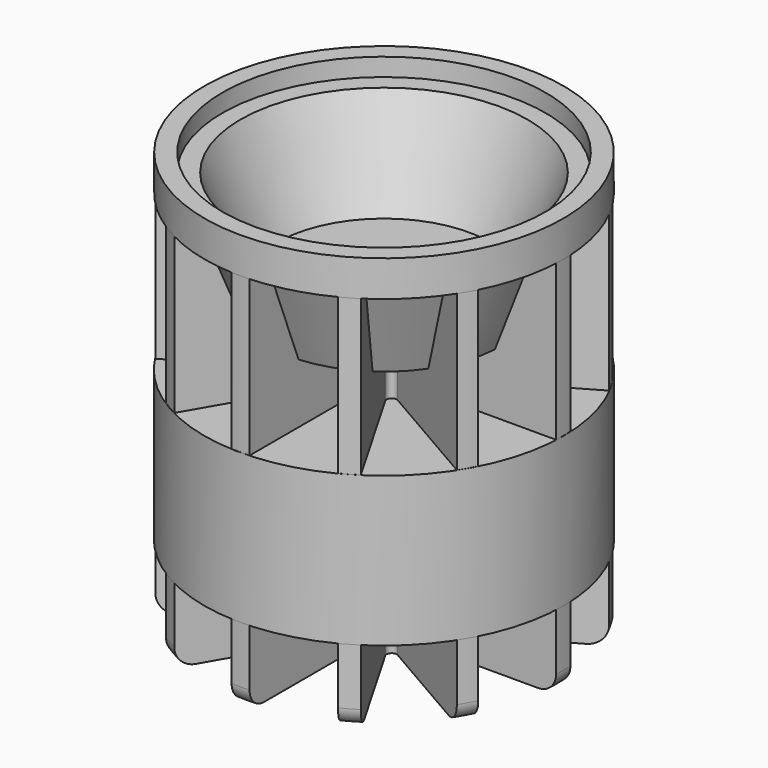
from build123d import *

# Parameters (mm, degrees)
F5_R     = 3
F7_R     = 30.0461893305
F8_DEPTH = 12.5


# Not quite as in the source:
# - after a boolean that leaves OpenCascade's solid faulty, fix() repairs it


with BuildPart() as f1:
    # F0 (on Right) → F1 (revolve)
    with BuildSketch(Plane.YZ):
        Polygon((-19.7913602038, -12.5343254842), (0, -12.5343254842), (0, -9.5343254842), (-17.7432774566, -9.5343254842), (-24, 6.4656745158), (-27, 6.4656745158), (-27, 9.4656745158), (-30, 9.4656745158), (-30, 3.4656745158), (-26.0480827472, 3.4656745158), align=None)
    revolve(axis=Axis((0, 0, -11.0343254842), (0, 0, -1)))

    # F3 (on offset) → F4 (join, up to the next surface of F1)
    with BuildSketch(Plane.XY.offset(-60)):
        with BuildLine():
            Line((-13.6822001609, -26.698265838), (-3.0822316874, -8.3385818833))
            ThreePointArc((-3.0822316874, -8.3385818833), (-2.1284587501, -7.9435161973), (-1.5, -8.7625395862))
            Line((-1.5, -8.7625395862), (-1.5, -29.9624765332))
            ThreePointArc((-1.5, -29.9624765332), (0, -30), (1.5, -29.9624765332))
            Line((1.5, -29.9624765332), (1.5, -8.7625395862))
            ThreePointArc((1.5, -8.7625395862), (2.1284587501, -7.9435161973), (3.0822316874, -8.3385818833))
            Line((3.0822316874, -8.3385818833), (13.6822001609, -26.698265838))
            ThreePointArc((13.6822001609, -26.698265838), (15, -25.9807621135), (16.2802763723, -25.198265838))
            Line((16.2802763723, -25.198265838), (5.6803078988, -6.8385818833))
            ThreePointArc((5.6803078988, -6.8385818833), (5.8150574471, -5.8150574471), (6.8385818833, -5.6803078988))
            Line((6.8385818833, -5.6803078988), (25.198265838, -16.2802763723))
            ThreePointArc((25.198265838, -16.2802763723), (25.9807621135, -15), (26.698265838, -13.6822001609))
            Line((26.698265838, -13.6822001609), (8.3385818833, -3.0822316874))
            ThreePointArc((8.3385818833, -3.0822316874), (7.9435161973, -2.1284587501), (8.7625395862, -1.5))
            Line((8.7625395862, -1.5), (29.9624765332, -1.5))
            ThreePointArc((29.9624765332, -1.5), (30, 0), (29.9624765332, 1.5))
            Line((29.9624765332, 1.5), (8.7625395862, 1.5))
            ThreePointArc((8.7625395862, 1.5), (7.9435161973, 2.1284587501), (8.3385818833, 3.0822316874))
            Line((8.3385818833, 3.0822316874), (26.698265838, 13.6822001609))
            ThreePointArc((26.698265838, 13.6822001609), (25.9807621135, 15), (25.198265838, 16.2802763723))
            Line((25.198265838, 16.2802763723), (6.8385818833, 5.6803078988))
            ThreePointArc((6.8385818833, 5.6803078988), (5.8150574471, 5.8150574471), (5.6803078988, 6.8385818833))
            Line((5.6803078988, 6.8385818833), (16.2802763723, 25.198265838))
            ThreePointArc((16.2802763723, 25.198265838), (15, 25.9807621135), (13.6822001609, 26.698265838))
            Line((13.6822001609, 26.698265838), (3.0822316874, 8.3385818833))
            ThreePointArc((3.0822316874, 8.3385818833), (2.1284587501, 7.9435161973), (1.5, 8.7625395862))
            Line((1.5, 8.7625395862), (1.5, 29.9624765332))
            ThreePointArc((1.5, 29.9624765332), (0, 30), (-1.5, 29.9624765332))
            Line((-1.5, 29.9624765332), (-1.5, 8.7625395862))
            ThreePointArc((-1.5, 8.7625395862), (-2.1284587501, 7.9435161973), (-3.0822316874, 8.3385818833))
            Line((-3.0822316874, 8.3385818833), (-13.6822001609, 26.698265838))
            ThreePointArc((-13.6822001609, 26.698265838), (-15, 25.9807621135), (-16.2802763723, 25.198265838))
            Line((-16.2802763723, 25.198265838), (-5.6803078988, 6.8385818833))
            ThreePointArc((-5.6803078988, 6.8385818833), (-5.8150574471, 5.8150574471), (-6.8385818833, 5.6803078988))
            Line((-6.8385818833, 5.6803078988), (-25.198265838, 16.2802763723))
            ThreePointArc((-25.198265838, 16.2802763723), (-25.9807621135, 15), (-26.698265838, 13.6822001609))
            Line((-26.698265838, 13.6822001609), (-8.3385818833, 3.0822316874))
            ThreePointArc((-8.3385818833, 3.0822316874), (-7.9435161973, 2.1284587501), (-8.7625395862, 1.5))
            Line((-8.7625395862, 1.5), (-29.9624765332, 1.5))
            ThreePointArc((-29.9624765332, 1.5), (-30, 0), (-29.9624765332, -1.5))
            Line((-29.9624765332, -1.5), (-8.7625395862, -1.5))
            ThreePointArc((-8.7625395862, -1.5), (-7.9435161973, -2.1284587501), (-8.3385818833, -3.0822316874))
            Line((-8.3385818833, -3.0822316874), (-26.698265838, -13.6822001609))
            ThreePointArc((-26.698265838, -13.6822001609), (-25.9807621135, -15), (-25.198265838, -16.2802763723))
            Line((-25.198265838, -16.2802763723), (-6.8385818833, -5.6803078988))
            ThreePointArc((-6.8385818833, -5.6803078988), (-5.8150574471, -5.8150574471), (-5.6803078988, -6.8385818833))
            Line((-5.6803078988, -6.8385818833), (-16.2802763723, -25.198265838))
            ThreePointArc((-16.2802763723, -25.198265838), (-15, -25.9807621135), (-13.6822001609, -26.698265838))
        make_face()
    extrude(until=Until.NEXT)

    add(f1.part.fix(), mode=Mode.REPLACE)

    # F5
    f5_edges = [f1.edges().sort_by_distance(p)[0] for p in [
        (-15, -25.980762, -60),
        (-25.980762, -15, -60),
        (-30, 0, -60),
        (-25.980762, 15, -60),
        (-15, 25.980762, -60),
        (0, 30, -60),
        (15, 25.980762, -60),
        (25.980762, 15, -60),
        (30, 0, -60),
        (25.980762, -15, -60),
        (15, -25.980762, -60),
        (0, -30, -60),
    ]]
    fillet(f5_edges, radius=F5_R)

    # F7 (on offset) → F8 (join, symmetric)
    with BuildSketch(Plane.XY.offset(-35)):
        Circle(F7_R)
    extrude(amount=F8_DEPTH, both=True)


solid = f1.part
